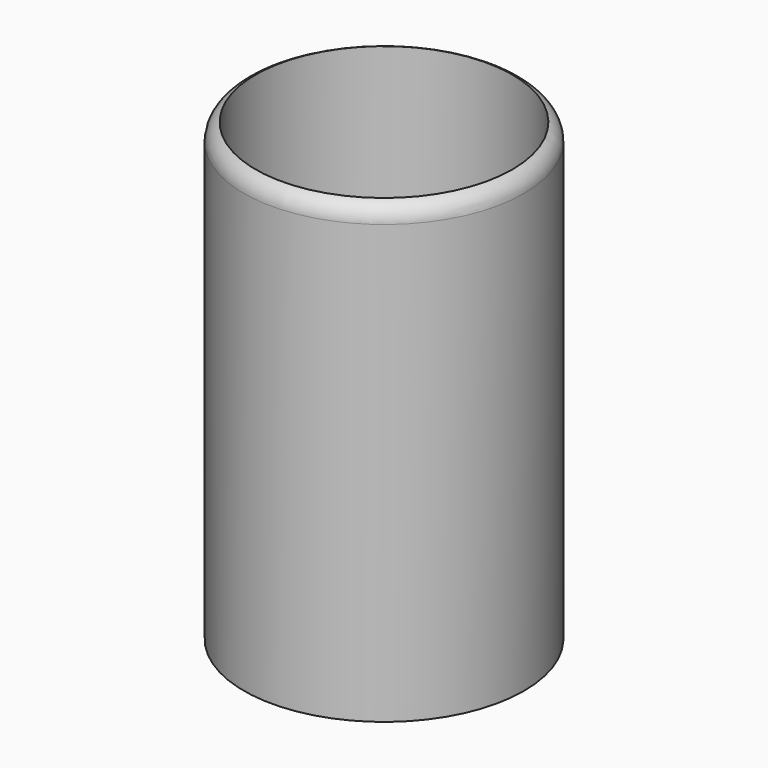
from build123d import *

# Parameters (mm, degrees)
F0_R     = 38.1
F0_R_2   = 34.925
F1_DEPTH = 73.025
F2_R     = 38.1
F2_R_2   = 33.3375
F3_DEPTH = 50.8


# Not quite as in the source:
# - a fillet or chamfer that OpenCascade refuses, or shapes differently, is made with other operations: its cross-section is extruded or revolved along the edge and cut away or added


with BuildPart() as f1:
    # F0 (on Top) → F1 (new body)
    with BuildSketch(Plane.XY):
        Circle(F0_R)
        Circle(F0_R_2, mode=Mode.SUBTRACT)
    extrude(amount=F1_DEPTH)

    # F2 (on Top) → F3 (join)
    with BuildSketch(Plane.XY):
        Circle(F2_R)
        Circle(F2_R_2, mode=Mode.SUBTRACT)
    extrude(amount=-F3_DEPTH)

    # F4: fillet of radius 5.08 on 1 edges, made by hand

    # F4_s1 → F4_t2 (revolve, cut)
    with BuildSketch(Plane.XZ):
        with BuildLine():
            ThreePointArc((38.1, 68.3157139607), (37.2321134838, 71.1555202921), (34.925, 73.025))
            Line((34.925, 73.025), (38.1, 73.025))
            Line((38.1, 73.025), (38.1, 68.3157139607))
        make_face()
    revolve(axis=Axis((0, 0, 73.025), (0, 0, 1)), mode=Mode.SUBTRACT)


solid = f1.part
